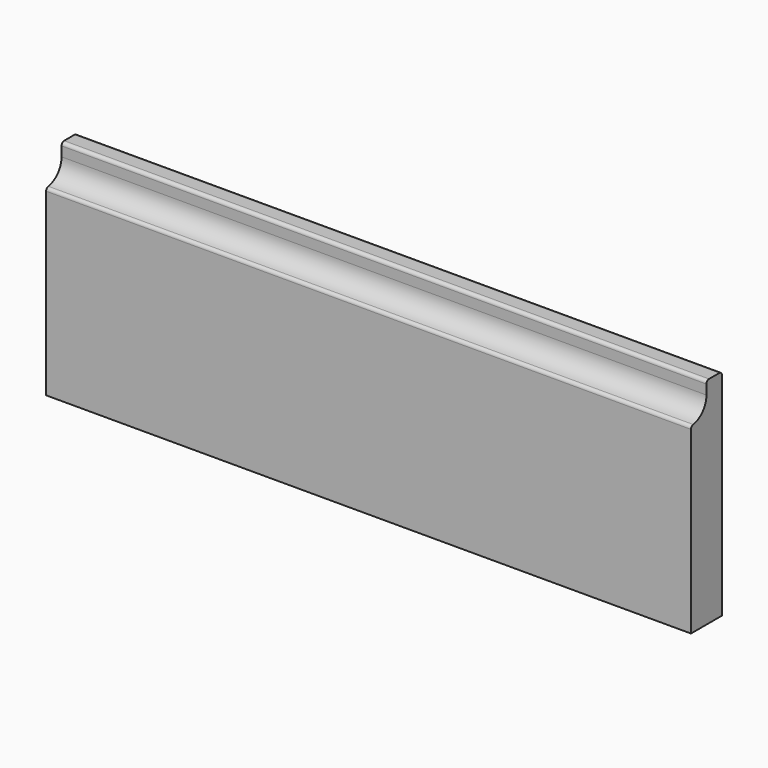
from build123d import *

# Parameters (mm, degrees)
F0_W     = 300
F0_H     = 100
F1_DEPTH = 9
F3_DEPTH = 300.001
F4_R     = 1.5


with BuildPart() as f1:
    # F0 (on Front) → F1 (new body, symmetric)
    with BuildSketch(Plane.XZ):
        with Locations((-3.7248600274, -105.7776198197)):
            Rectangle(F0_W, F0_H)
    extrude(amount=F1_DEPTH, both=True)

    # F2 (on face) → F3 (cut, through all)
    with BuildSketch(Plane.YZ.offset(146.2751399726)):
        with BuildLine():
            Line((0, -61.7776198197), (0, -55.7776198197))
            Line((0, -55.7776198197), (-9, -55.7776198197))
            Line((-9, -55.7776198197), (-9, -70.7776198197))
            ThreePointArc((-9, -70.7776198197), (-2.6360389693, -68.1415808503), (0, -61.7776198197))
        make_face()
    extrude(amount=-F3_DEPTH, mode=Mode.SUBTRACT)

    # F4
    f4_edges = [f1.edges().sort_by_distance(p)[0] for p in [
        (-3.72486, 0, -55.77762),
        (-3.72486, 9, -55.77762),
        (-3.72486, -9, -70.77762),
    ]]
    fillet(f4_edges, radius=F4_R)


solid = f1.part
